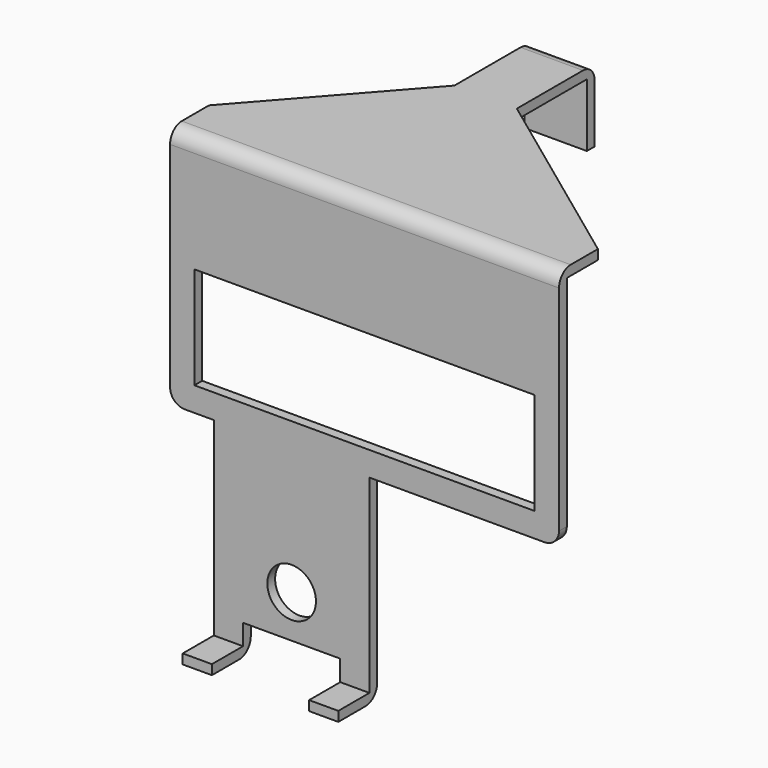
from build123d import *

# Parameters (mm, degrees)
F0_R     = 5
F0_W     = 70
F0_H     = 21
F1_DEPTH = 2
F2_W     = 6
F2_H     = 2
F3_DEPTH = 8
F4_R     = 3
F6_DEPTH = 2
F7_W     = 12.8450786794
F7_H     = 2
F8_DEPTH = 13
F9_R     = 3


with BuildPart() as f1:
    # F0 (on Front) → F1 (new body)
    with BuildSketch(Plane.XZ):
        with BuildLine():
            Line((28.9647261798, 43.8778921962), (-51.0352738202, 43.8778921962))
            Line((-51.0352738202, 43.8778921962), (-51.0352738202, -3.1221078038))
            ThreePointArc((-51.0352738202, -3.1221078038), (-50.1565941637, -5.2434281474), (-48.0352738202, -6.1221078038))
            Line((-48.0352738202, -6.1221078038), (-42.0352738202, -6.1221078038))
            Line((-42.0352738202, -6.1221078038), (-42.0352738202, -47.1221078038))
            Line((-42.0352738202, -47.1221078038), (-36.0352738202, -47.1221078038))
            Line((-36.0352738202, -47.1221078038), (-36.0352738202, -40.8721078038))
            Line((-36.0352738202, -40.8721078038), (-16.0352738202, -40.8721078038))
            Line((-16.0352738202, -40.8721078038), (-16.0352738202, -47.1221078038))
            Line((-16.0352738202, -47.1221078038), (-10.0352738202, -47.1221078038))
            Line((-10.0352738202, -47.1221078038), (-10.0352738202, -6.1221078038))
            Line((-10.0352738202, -6.1221078038), (25.9647261798, -6.1221078038))
            ThreePointArc((25.9647261798, -6.1221078038), (28.0860465234, -5.2434281474), (28.9647261798, -3.1221078038))
            Line((28.9647261798, -3.1221078038), (28.9647261798, 43.8778921962))
        make_face()
        with Locations((-26.0352738202, -32.1221078038)):
            Circle(F0_R, mode=Mode.SUBTRACT)
        with Locations((-11.0352738202, 9.3778921962)):
            Rectangle(F0_W, F0_H, mode=Mode.SUBTRACT)
    extrude(amount=F1_DEPTH)

    # F2 (on face) → F3 (join)
    with BuildSketch(Plane.XZ.offset(2)):
        with Locations((-39.0352738202, -46.1221078038)):
            Rectangle(F2_W, F2_H)
        with Locations((-13.0352738202, -46.1221078038)):
            Rectangle(F2_W, F2_H)
    extrude(amount=F3_DEPTH)

    # F4
    f4_edges = [f1.edges().sort_by_distance(p)[0] for p in [
        (-13.035274, 0, -47.122108),
        (-39.035274, 0, -47.122108),
    ]]
    fillet(f4_edges, radius=F4_R)

    # F5 (on face) → F6 (join)
    with BuildSketch(Plane.XY.offset(43.8778921962)):
        Polygon((-51.0352738202, 8), (-51.0352738202, 0), (28.9647261798, 0), (28.9647261798, 8), (-11.7104330932, 38), (-11.7104330932, 58), (-24.5555117726, 58), (-24.5555117726, 38), align=None)
    extrude(amount=-F6_DEPTH)

    # F7 (on face) → F8 (join)
    with BuildSketch(Plane(origin=(0, 0, 41.8778921962), x_dir=(1, 0, 0), z_dir=(0, 0, -1))):
        with Locations((-18.1329724329, -57)):
            Rectangle(F7_W, F7_H)
    extrude(amount=F8_DEPTH)

    # F9
    f9_edges = [f1.edges().sort_by_distance(p)[0] for p in [
        (-18.132972, 58, 43.877892),
        (-11.035274, -2, 43.877892),
    ]]
    fillet(f9_edges, radius=F9_R)


solid = f1.part
